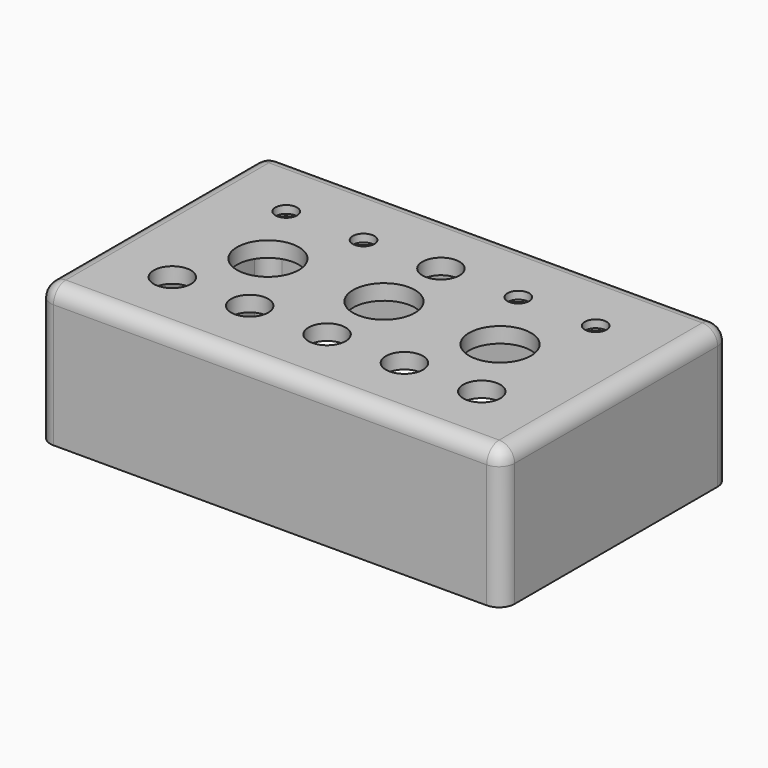
from build123d import *

# Parameters (mm, degrees)
F0_W         = 150
F0_H         = 92
F0_R         = 6
F0_R_2       = 10
F0_R_3       = 3.5
F1_DEPTH     = 2.5
F2_W         = 150
F2_H         = 92
F2_R         = 6
F2_R_2       = 10
F2_R_3       = 7
F3_DEPTH     = 2.5
F4_R         = 4.99999
F5_W         = 150
F5_H         = 92
F6_DEPTH     = 40
F7_T1_DEPTH  = 57.5
F7_T4_ANGLE  = 90
F7_T6_ANGLE  = 90
F7_T8_ANGLE  = 90
F7_T10_ANGLE = 90


# Not quite as in the source:
# - a fillet or chamfer that OpenCascade refuses, or shapes differently, is made with other operations: its cross-section is extruded or revolved along the edge and cut away or added
# - a fillet or chamfer is up to 0.001 mm smaller than in the source, because OpenCascade refuses the exact size


with BuildPart() as f1:
    # F0 (on Top) → F1 (new body)
    with BuildSketch(Plane.XY):
        Rectangle(F0_W, F0_H)
        with Locations((-50, -23)):
            Circle(F0_R, mode=Mode.SUBTRACT)
        with Locations((-25, -23)):
            Circle(F0_R, mode=Mode.SUBTRACT)
        with Locations((0, -23)):
            Circle(F0_R, mode=Mode.SUBTRACT)
        with Locations((25, -23)):
            Circle(F0_R, mode=Mode.SUBTRACT)
        with Locations((50, -23)):
            Circle(F0_R, mode=Mode.SUBTRACT)
        with Locations((-37.5, 0)):
            Circle(F0_R_2, mode=Mode.SUBTRACT)
        with Locations((-50, 23)):
            Circle(F0_R_3, mode=Mode.SUBTRACT)
        with Locations((-25, 23)):
            Circle(F0_R_3, mode=Mode.SUBTRACT)
        Circle(F0_R_2, mode=Mode.SUBTRACT)
        with Locations((37.5, 0)):
            Circle(F0_R_2, mode=Mode.SUBTRACT)
        with Locations((0, 23)):
            Circle(F0_R, mode=Mode.SUBTRACT)
        with Locations((25, 23)):
            Circle(F0_R_3, mode=Mode.SUBTRACT)
        with Locations((50, 23)):
            Circle(F0_R_3, mode=Mode.SUBTRACT)
    extrude(amount=F1_DEPTH)

    # F2 (on Top) → F3 (join)
    with BuildSketch(Plane.XY):
        Rectangle(F2_W, F2_H)
        with Locations((-50, -23)):
            Circle(F2_R, mode=Mode.SUBTRACT)
        with Locations((-25, -23)):
            Circle(F2_R, mode=Mode.SUBTRACT)
        with Locations((0, -23)):
            Circle(F2_R, mode=Mode.SUBTRACT)
        with Locations((25, -23)):
            Circle(F2_R, mode=Mode.SUBTRACT)
        with Locations((50, -23)):
            Circle(F2_R, mode=Mode.SUBTRACT)
        with Locations((-37.5, 0)):
            Circle(F2_R_2, mode=Mode.SUBTRACT)
        with Locations((-50, 23)):
            Circle(F2_R_3, mode=Mode.SUBTRACT)
        with Locations((-25, 23)):
            Circle(F2_R_3, mode=Mode.SUBTRACT)
        Circle(F2_R_2, mode=Mode.SUBTRACT)
        with Locations((37.5, 0)):
            Circle(F2_R_2, mode=Mode.SUBTRACT)
        with Locations((0, 23)):
            Circle(F2_R, mode=Mode.SUBTRACT)
        with Locations((25, 23)):
            Circle(F2_R_3, mode=Mode.SUBTRACT)
        with Locations((50, 23)):
            Circle(F2_R_3, mode=Mode.SUBTRACT)
    extrude(amount=-F3_DEPTH)

    # F4 (radius 5 in the source; OpenCascade refuses exactly that, so slightly less here)
    f4_edges = [f1.edges().sort_by_distance(p)[0] for p in [
        (0, 46, 2.5),
        (-75, 0, 2.5),
        (0, -46, 2.5),
        (75, 0, 2.5),
    ]]
    fillet(f4_edges, radius=F4_R)

    # F5 (on face) → F6 (join)
    with BuildSketch(Plane(origin=(0, 0, -2.5), x_dir=(1, 0, 0), z_dir=(0, 0, -1))):
        Rectangle(F5_W, F5_H)
        with BuildLine():
            ThreePointArc((-73.5, 39.5), (-72.0355339059, 43.0355339059), (-68.5, 44.5))
            Line((-68.5, 44.5), (68.5, 44.5))
            ThreePointArc((68.5, 44.5), (72.0355339059, 43.0355339059), (73.5, 39.5))
            Line((73.5, 39.5), (73.5, -39.5))
            ThreePointArc((73.5, -39.5), (72.0355339059, -43.0355339059), (68.5, -44.5))
            Line((68.5, -44.5), (-68.5, -44.5))
            ThreePointArc((-68.5, -44.5), (-72.0355339059, -43.0355339059), (-73.5, -39.5))
            Line((-73.5, -39.5), (-73.5, 39.5))
        make_face(mode=Mode.SUBTRACT)
    extrude(amount=F6_DEPTH)

    # F7: fillet of radius 5 on 4 edges, made by hand

    # F7_s2 → F7_t1 (cut)
    with BuildSketch(Plane.XY.offset(-55)):
        with BuildLine():
            ThreePointArc((70, -46), (73.5355339059, -44.5355339059), (75, -41))
            Line((75, -41), (75, -46))
            Line((75, -46), (70, -46))
        make_face()
        with BuildLine():
            ThreePointArc((70, 46), (73.5355339059, 44.5355339059), (75, 41))
            Line((75, 41), (75, 46))
            Line((75, 46), (70, 46))
        make_face()
        with BuildLine():
            ThreePointArc((-70, 46), (-73.5355339059, 44.5355339059), (-75, 41))
            Line((-75, 41), (-75, 46))
            Line((-75, 46), (-70, 46))
        make_face()
        with BuildLine():
            ThreePointArc((-70, -46), (-73.5355339059, -44.5355339059), (-75, -41))
            Line((-75, -41), (-75, -46))
            Line((-75, -46), (-70, -46))
        make_face()
    extrude(amount=F7_T1_DEPTH, mode=Mode.SUBTRACT)

    # F7_s3 → F7_t4 (revolve, cut)
    with BuildSketch(Plane.XZ.offset(41)):
        with BuildLine():
            ThreePointArc((-70.00001, 2.5), (-73.5355368349, 1.0355368349), (-75, -2.49999))
            Line((-75, -2.49999), (-75, 2.5))
            Line((-75, 2.5), (-70.00001, 2.5))
        make_face()
    revolve(axis=Axis((-70, -41, 2.5), (0, 0, 1)), revolution_arc=F7_T4_ANGLE, mode=Mode.SUBTRACT)

    # F7_s5 → F7_t6 (revolve, cut)
    with BuildSketch(Plane.YZ.offset(-70)):
        with BuildLine():
            ThreePointArc((41.00001, 2.5), (44.5355368349, 1.0355368349), (46, -2.49999))
            Line((46, -2.49999), (46, 2.5))
            Line((46, 2.5), (41.00001, 2.5))
        make_face()
    revolve(axis=Axis((-70, 41, 2.5), (0, 0, 1)), revolution_arc=F7_T6_ANGLE, mode=Mode.SUBTRACT)

    # F7_s7 → F7_t8 (revolve, cut)
    with BuildSketch(Plane.XZ.offset(-41)):
        with BuildLine():
            ThreePointArc((70.00001, 2.5), (73.5355368349, 1.0355368349), (75, -2.49999))
            Line((75, -2.49999), (75, 2.5))
            Line((75, 2.5), (70.00001, 2.5))
        make_face()
    revolve(axis=Axis((70, 41, 2.5), (0, 0, 1)), revolution_arc=F7_T8_ANGLE, mode=Mode.SUBTRACT)

    # F7_s9 → F7_t10 (revolve, cut)
    with BuildSketch(Plane.YZ.offset(70)):
        with BuildLine():
            ThreePointArc((-41.00001, 2.5), (-44.5355368349, 1.0355368349), (-46, -2.49999))
            Line((-46, -2.49999), (-46, 2.5))
            Line((-46, 2.5), (-41.00001, 2.5))
        make_face()
    revolve(axis=Axis((70, -41, 2.5), (0, 0, 1)), revolution_arc=F7_T10_ANGLE, mode=Mode.SUBTRACT)


solid = f1.part
